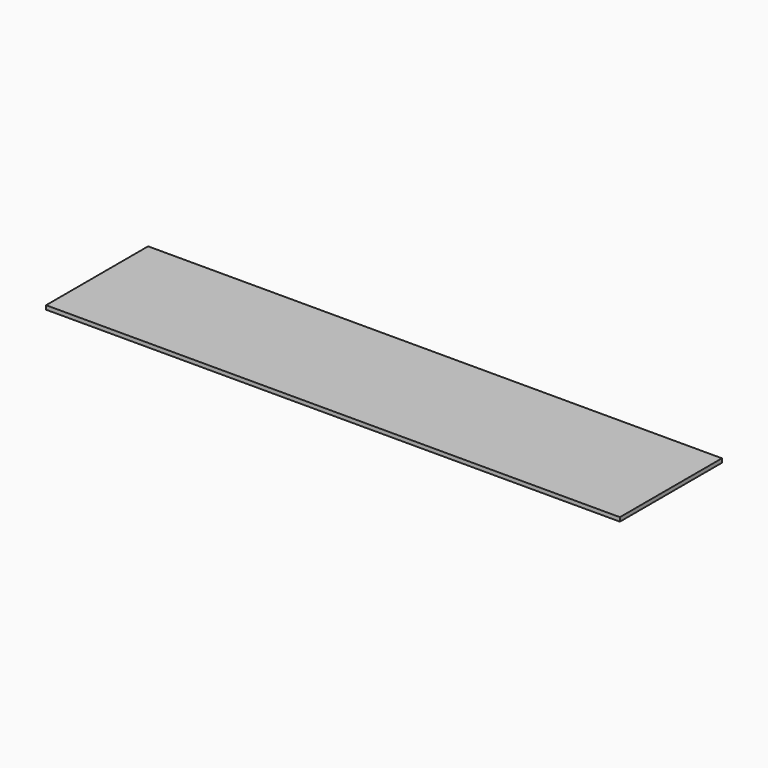
from build123d import *

# Parameters (mm, degrees)
F1_W     = 2743.2
F1_H     = 609.6
F2_DEPTH = 19.05


# Not quite as in the source:
# - a variable given as a bare number and used for a length is read in inches; the dataset says mm whatever the document's units were


with BuildPart() as f2:
    # F1 (on Top) → F2 (new body)
    with BuildSketch(Plane.XY):
        Rectangle(F1_W, F1_H)
    extrude(amount=-F2_DEPTH)


solid = f2.part
